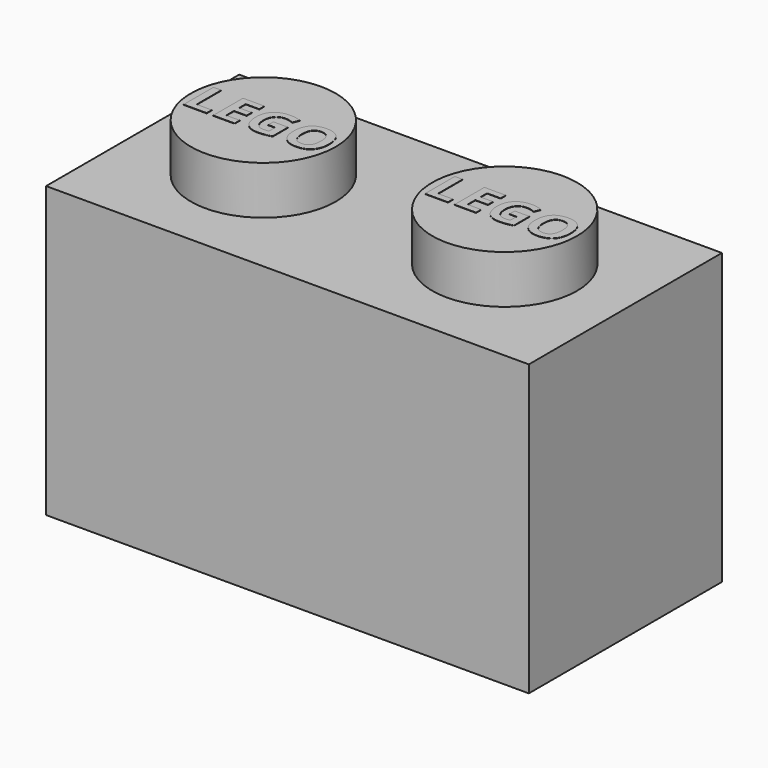
from build123d import *

# Parameters (mm, degrees)
F0_W         = 16
F0_H         = 8
F1_DEPTH     = 9.6
F2_W         = 12.8
F2_H         = 4.8
F3_DEPTH     = 8
F4_R         = 1.6
F5_DEPTH     = 1.6
F6_R         = 2.4
F7_DEPTH     = 1.6
F8_TEXT_SIZE = 1.7347239408
F9_DEPTH     = 0.01


# Not quite as in the source:
# - Text() gives the source's letters only with a copy of the font that has no kerning and outlines rounded to 1/6400 em; it was checked with that copy


with BuildPart() as f1:
    # F0 (on Top) → F1 (new body)
    with BuildSketch(Plane.XY):
        Rectangle(F0_W, F0_H)
    extrude(amount=F1_DEPTH)

    # F2 (on face) → F3 (cut)
    with BuildSketch(Plane(origin=(0, 0, 0), x_dir=(1, 0, 0), z_dir=(0, 0, -1))):
        Rectangle(F2_W, F2_H)
    extrude(amount=-F3_DEPTH, mode=Mode.SUBTRACT)

    # F4 (on face) → F5 (cut)
    with BuildSketch(Plane(origin=(0, 0, 8), x_dir=(1, 0, 0), z_dir=(0, 0, -1))):
        with Locations((-4, 0)):
            Circle(F4_R)
        with Locations((4, 0)):
            Circle(F4_R)
    extrude(amount=-F5_DEPTH, mode=Mode.SUBTRACT)

    # F6 (on face) → F7 (join)
    with BuildSketch(Plane.XY.offset(9.6)):
        with Locations((-4, 0)):
            Circle(F6_R)
        with Locations((4, 0)):
            Circle(F6_R)
    extrude(amount=F7_DEPTH)

    # F8 (on face) → F9 (join)
    with BuildSketch(Plane.XY.offset(11.2)):
        with Locations((-6.3, -0.6245012374)):
            Text('LEGO', F8_TEXT_SIZE, font='Open Sans', font_style=FontStyle.BOLD, text_align=(TextAlign.LEFT, TextAlign.BOTTOM))
        with Locations((1.7, -0.6245)):
            Text('LEGO', F8_TEXT_SIZE, font='Open Sans', font_style=FontStyle.BOLD, text_align=(TextAlign.LEFT, TextAlign.BOTTOM))
    extrude(amount=F9_DEPTH)


solid = f1.part
